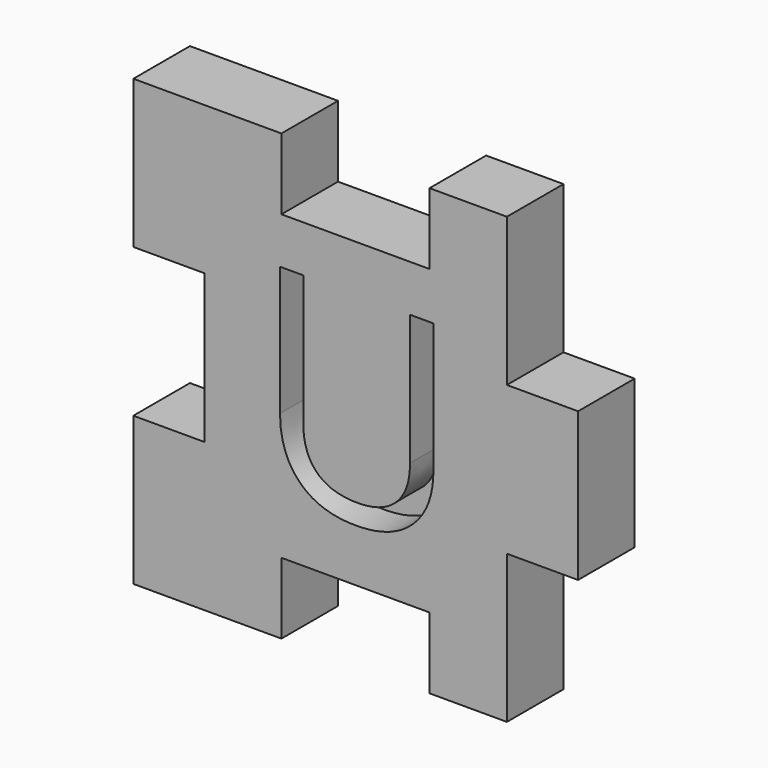
from build123d import *

# Parameters (mm, degrees)
F1_DEPTH     = 2.032
F2_TEXT_SIZE = 8.0645199199
F3_DEPTH     = 1


# Not quite as in the source:
# - a length typed as a fraction of an inch, garbled in the dataset ("3 / 203.2 mm" for 3/8 in), is restored
# - Text() gives the source's letters only with a copy of the font that has no kerning and outlines rounded to 1/6400 em; it was checked with that copy


with BuildPart() as f1:
    # F0 (on Front) → F1 (new body)
    with BuildSketch(Plane.XZ):
        Polygon((-10.9897290399, 29.0234165891), (-10.9897290399, 26.8898165891), (-10.9897290399, 24.7562165891), (-13.0344290399, 24.7562165891), (-13.0344290399, 20.5017165891), (-8.7799290399, 20.5017165891), (-8.7799290399, 22.5464165891), (-4.5254290399, 22.5464165891), (-4.5254290399, 20.5017165891), (-2.3029290399, 20.5017165891), (-2.3029290399, 24.7562165891), (-0.2582290399, 24.7562165891), (-0.2582290399, 29.0234165891), (-2.3029290399, 29.0234165891), (-2.3029290399, 33.2779165891), (-4.5254290399, 33.2779165891), (-4.5254290399, 31.2332165891), (-8.7799290399, 31.2332165891), (-8.7799290399, 33.2779165891), (-13.0344290399, 33.2779165891), (-13.0344290399, 29.0234165891), align=None)
    extrude(amount=F1_DEPTH)

    # F2 (on face) → F3 (cut)
    with BuildSketch(Plane.XZ.offset(2.032)):
        with Locations((-9.5529981592, 24.1369831498)):
            Text('U', F2_TEXT_SIZE, font='Open Sans', text_align=(TextAlign.LEFT, TextAlign.BOTTOM))
    extrude(amount=-F3_DEPTH, mode=Mode.SUBTRACT)


solid = f1.part
